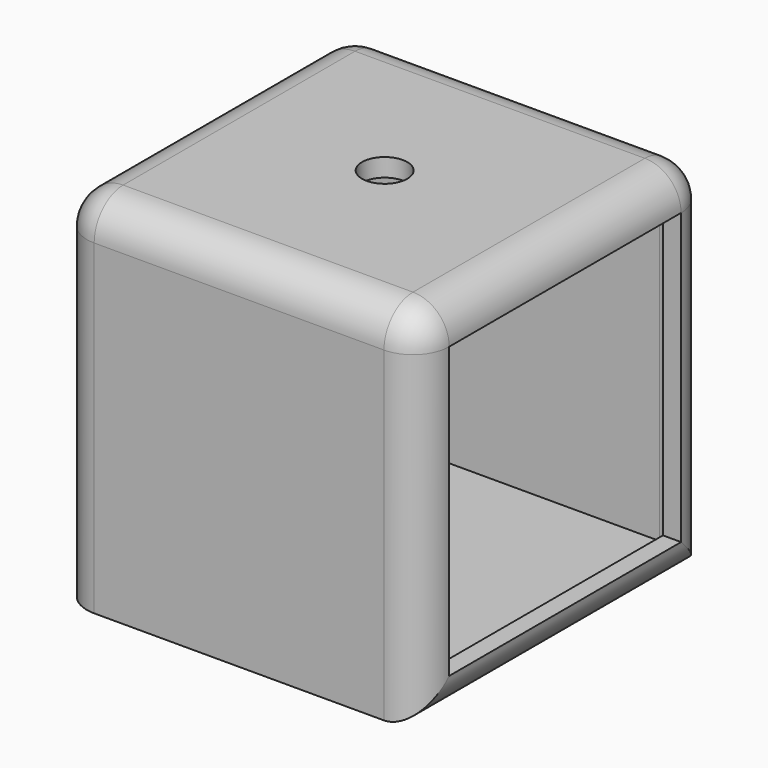
from build123d import *

# Parameters (mm, degrees)
F0_W     = 50.8
F0_H     = 50.8
F1_DEPTH = 50.8
F3_R     = 5.08
F5_T     = -2.54
F7_D     = 6.35


# Not quite as in the source:
# - a shell that OpenCascade refuses in one call is made with other operations: the cavity is built on its own and cut out


with BuildPart() as f1:
    # F0 (on Top) → F1 (new body)
    with BuildSketch(Plane.XY):
        with Locations((-29.015717721, -32.2184429228)):
            Rectangle(F0_W, F0_H)
    extrude(amount=F1_DEPTH)

    # F3
    f3_edges = [f1.edges().sort_by_distance(p)[0] for p in [
        (-29.015718, -57.618443, 50.8),
        (-54.415718, -32.218443, 50.8),
        (-29.015718, -6.818443, 50.8),
        (-3.615718, -32.218443, 50.8),
        (-54.415718, -57.618443, 25.4),
        (-54.415718, -6.818443, 25.4),
        (-3.615718, -6.818443, 25.4),
        (-3.615718, -57.618443, 25.4),
        (-3.615718, -32.218443, 0),
    ]]
    fillet(f3_edges, radius=F3_R)

    # F5: a shell. OpenCascade refuses it in one call, so the cavity is built on its own and cut out:
    # the body offset inwards by the wall thickness, plus a prism from it out through each open face.
    f5_core = offset(f1.part, amount=F5_T, mode=Mode.PRIVATE)
    f5_exits = [f5_core.faces().sort_by_distance(p)[0] for p in [
        (-6.155718, -32.218443, 25.4),
    ]]
    add(f5_core, mode=Mode.SUBTRACT)
    extrude(f5_exits, amount=-F5_T, mode=Mode.SUBTRACT)

    # F7 (through all)
    with Locations(Plane.XY.offset(50.8)):
        with Locations((-29.1464701295, -31.9354347885)):
            Hole(F7_D / 2)


solid = f1.part
